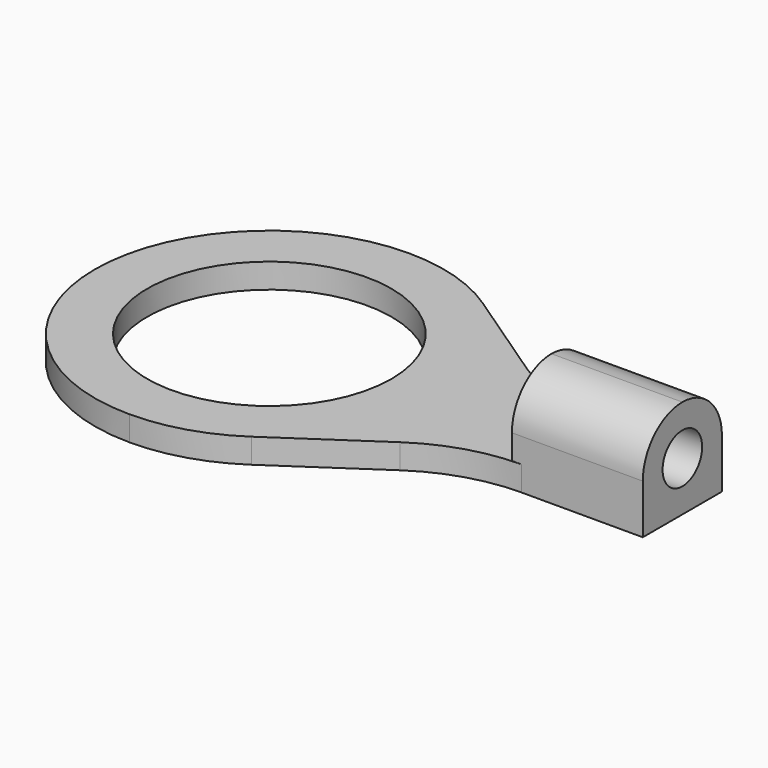
from build123d import *

# Parameters (mm, degrees)
F0_R     = 4.2
F1_DEPTH = 0.85
F3_DEPTH = 2.55
F4_R     = 1.69999
F5_R     = 0.85
F6_DEPTH = 25


# Not quite as in the source:
# - a fillet or chamfer is up to 0.001 mm smaller than in the source, because OpenCascade refuses the exact size


with BuildPart() as f1:
    # F0 (on Top) → F1 (new body)
    with BuildSketch(Plane.XY):
        with BuildLine():
            Line((16.0373335058, 4.3), (20.2, 4.3))
            Line((20.2, 4.3), (20.2, 7.7))
            Line((20.2, 7.7), (16.0373335058, 7.7))
            ThreePointArc((16.0373335058, 7.7), (14.2805243712, 7.9629605488), (12.6777057346, 8.7287927785))
            Line((12.6777057346, 8.7287927785), (9.3596277711, 10.9712072215))
            ThreePointArc((9.3596277711, 10.9712072215), (7.7568091346, 11.7370394512), (6, 12))
            ThreePointArc((6, 12), (1.7573593129, 10.2426406871), (0, 6))
            ThreePointArc((0, 6), (1.7573593129, 1.7573593129), (6, 0))
            ThreePointArc((6, 0), (7.7568091346, 0.2629605488), (9.3596277711, 1.0287927785))
            Line((9.3596277711, 1.0287927785), (12.6777057346, 3.2712072215))
            ThreePointArc((12.6777057346, 3.2712072215), (14.2805243712, 4.0370394512), (16.0373335058, 4.3))
        make_face()
        with Locations((6, 6)):
            Circle(F0_R, mode=Mode.SUBTRACT)
    extrude(amount=F1_DEPTH)

    # F2 (on face) → F3 (join)
    with BuildSketch(Plane.XY.offset(0.85)):
        Polygon((20.2, 4.3), (20.2, 7.7), (16.0373335058, 7.7), (15.7, 7.7), (15.7, 4.3), (16.0373335058, 4.3), align=None)
    extrude(amount=F3_DEPTH)

    # F4 (radius 1.7 in the source; OpenCascade refuses exactly that, so slightly less here)
    f4_edges = [f1.edges().sort_by_distance(p)[0] for p in [
        (17.95, 7.7, 3.4),
        (17.95, 4.3, 3.4),
    ]]
    fillet(f4_edges, radius=F4_R)

    # F5 (on face) → F6 (cut)
    with BuildSketch(Plane.YZ.offset(20.2)):
        with Locations((6, 1.7)):
            Circle(F5_R)
    extrude(amount=-F6_DEPTH, mode=Mode.SUBTRACT)


solid = f1.part
